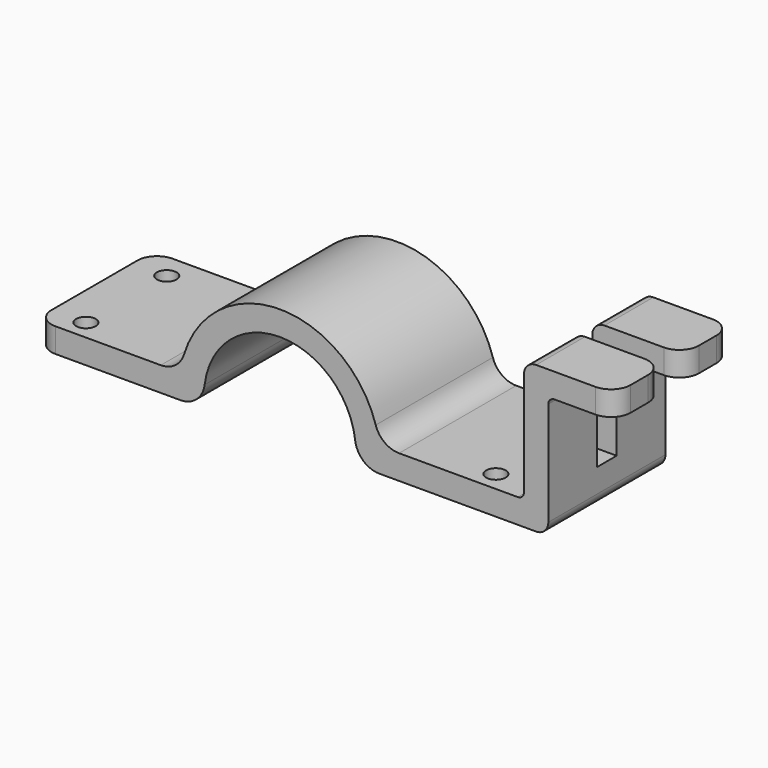
from build123d import *

# Parameters (mm, degrees)
F1_DEPTH = 19.05
F2_W     = 6.35
F2_H     = 28.8036865525
F3_DEPTH = 25.4
F4_R     = 5.08
F6_D     = 5.1054


# Not quite as in the source:
# - a feature names something its author has since deleted; it is built from what else it names


with BuildPart() as f1:
    # F0 (on Front) → F1 (new body, symmetric)
    with BuildSketch(Plane.XZ):
        with BuildLine():
            Line((-63.5, 3.175), (-63.5, -3.175))
            Line((-63.5, -3.175), (-25.8909725642, -3.175))
            ThreePointArc((-25.8909725642, -3.175), (-21.6829722848, -1.5805476707), (-19.5881864455, 2.4020917642))
            ThreePointArc((-19.5881864455, 2.4020917642), (0, 19.7349206501), (19.5881864455, 2.4020917642))
            ThreePointArc((19.5881864455, 2.4020917642), (21.6829722848, -1.5805476707), (25.8909725642, -3.175))
            Line((25.8909725642, -3.175), (63.5, -3.175))
            Line((63.5, -3.175), (66.675, -3.175))
            ThreePointArc((66.675, -3.175), (68.9200640303, -2.2450640303), (69.85, 0))
            Line((69.85, 0), (69.85, 27.0641443402))
            ThreePointArc((69.85, 27.0641443402), (70.3149679849, 28.1866763553), (71.4375, 28.6516443402))
            Line((71.4375, 28.6516443402), (87.1900793672, 28.6516443402))
            Line((87.1900793672, 28.6516443402), (87.1900793672, 35.0016443402))
            Line((87.1900793672, 35.0016443402), (66.675, 35.0016443402))
            ThreePointArc((66.675, 35.0016443402), (64.4299359697, 34.0717083704), (63.5, 31.8266443402))
            Line((63.5, 31.8266443402), (63.5, 4.7625))
            ThreePointArc((63.5, 4.7625), (63.0350320151, 3.6399679849), (61.9125, 3.175))
            Line((61.9125, 3.175), (31.0048133776, 3.175))
            ThreePointArc((31.0048133776, 3.175), (27.2311418069, 4.4179555635), (24.9347949838, 7.6602274404))
            ThreePointArc((24.9347949838, 7.6602274404), (0, 26.0849206501), (-24.9347949838, 7.6602274404))
            ThreePointArc((-24.9347949838, 7.6602274404), (-27.2311418069, 4.4179555635), (-31.0048133776, 3.175))
            Line((-31.0048133776, 3.175), (-63.5, 3.175))
        make_face()
    extrude(amount=F1_DEPTH, both=True)

    # F2 (on face) → F3 (cut)
    with BuildSketch(Plane.YZ.offset(87.1900793672)):
        with Locations((0, 20.5998010639)):
            Rectangle(F2_W, F2_H)
    extrude(amount=-F3_DEPTH, mode=Mode.SUBTRACT)

    # F4
    f4_edges = [f1.edges().sort_by_distance(p)[0] for p in [
        (-63.5, -19.05, 0),
        (-63.5, 19.05, 0),
        (87.190079, 19.05, 31.826644),
        (87.190079, 3.175, 31.826644),
        (87.190079, -3.175, 31.826644),
        (87.190079, -19.05, 31.826644),
    ]]
    fillet(f4_edges, radius=F4_R)

    # F6 (through all)
    with Locations(Plane.XY.offset(3.175)):
        with Locations((-54.6063743532, 12.3959155753), (-54.6063743532, -13.8984508812), (52.6370815933, 12.3959155753), (52.0736314356, -13.8984508812)):
            Hole(F6_D / 2)


solid = f1.part
